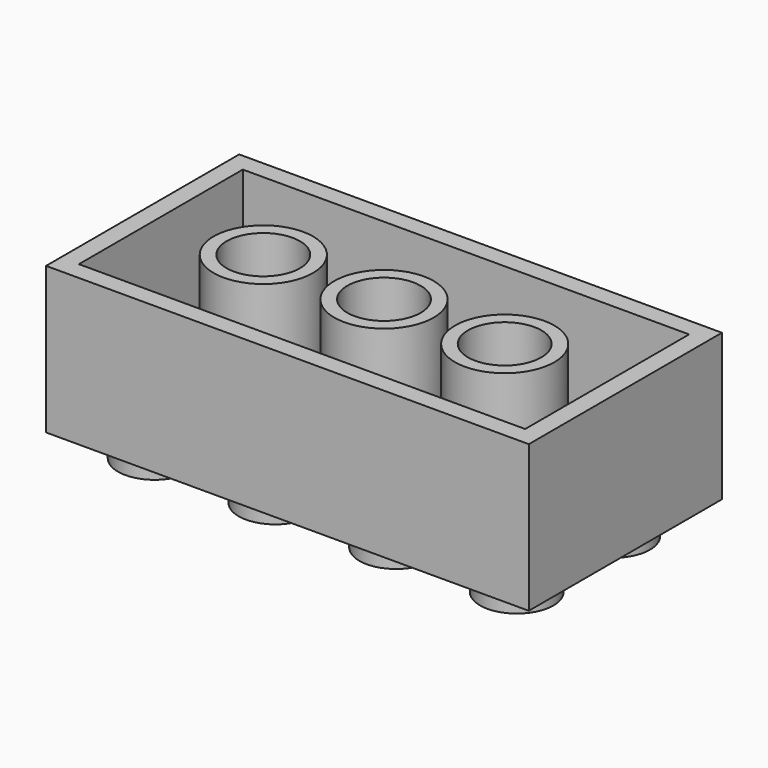
from build123d import *

# Parameters (mm, degrees)
F0_R     = 2.4003
F1_DEPTH = 9.6012
F2_DEPTH = 1.8034
F3_T     = -1.1938
F4_R     = 3.2512
F4_R_2   = 2.4003
F5_DEPTH = 9.6012


# Not quite as in the source:
# - a feature names something its author has since deleted; it is built from what else it names


with BuildPart() as f1:
    # F0 (on Top) → F1 (new body)
    with BuildSketch(Plane.XY):
        Polygon((-11.8491, 16.497923825), (-11.8491, 8.598523825), (-11.8491, 0.699123825), (-3.9497, 0.699123825), (3.9497, 0.699123825), (11.8491, 0.699123825), (19.7485, 0.699123825), (19.7485, 8.598523825), (19.7485, 16.497923825), (11.8491, 16.497923825), (3.9497, 16.497923825), (-3.9497, 16.497923825), align=None)
        with Locations((-7.8994, 4.648823825)):
            Circle(F0_R, mode=Mode.SUBTRACT)
        with Locations((0, 4.648823825)):
            Circle(F0_R, mode=Mode.SUBTRACT)
        with Locations((7.8994, 4.648823825)):
            Circle(F0_R, mode=Mode.SUBTRACT)
        with Locations((15.7988, 4.648823825)):
            Circle(F0_R, mode=Mode.SUBTRACT)
        with Locations((-7.8994, 12.548223825)):
            Circle(F0_R, mode=Mode.SUBTRACT)
        with Locations((0, 12.548223825)):
            Circle(F0_R, mode=Mode.SUBTRACT)
        with Locations((7.8994, 12.548223825)):
            Circle(F0_R, mode=Mode.SUBTRACT)
        with Locations((15.7988, 12.548223825)):
            Circle(F0_R, mode=Mode.SUBTRACT)
        with Locations((-7.8994, 4.648823825)):
            Circle(F0_R)
        with Locations((-7.8994, 12.548223825)):
            Circle(F0_R)
        with Locations((0, 4.648823825)):
            Circle(F0_R)
        with Locations((0, 12.548223825)):
            Circle(F0_R)
        with Locations((7.8994, 4.648823825)):
            Circle(F0_R)
        with Locations((15.7988, 4.648823825)):
            Circle(F0_R)
        with Locations((15.7988, 12.548223825)):
            Circle(F0_R)
        with Locations((7.8994, 12.548223825)):
            Circle(F0_R)
    extrude(amount=F1_DEPTH)

    # F3
    f3_openings = [f1.faces().sort_by_distance(p)[0] for p in [
        (3.9497, 8.598524, 9.6012),
    ]]
    offset(amount=F3_T, openings=f3_openings)

    # F4 (on face) → F5 (join)
    with BuildSketch(Plane.XY.offset(9.6012)):
        with Locations((-3.9497, 8.598523825)):
            Circle(F4_R)
        with Locations((-3.9497, 8.598523825)):
            Circle(F4_R_2, mode=Mode.SUBTRACT)
        with Locations((3.9497, 8.598523825)):
            Circle(F4_R)
        with Locations((3.9497, 8.598523825)):
            Circle(F4_R_2, mode=Mode.SUBTRACT)
        with Locations((11.8491, 8.598523825)):
            Circle(F4_R)
        with Locations((11.8491, 8.598523825)):
            Circle(F4_R_2, mode=Mode.SUBTRACT)
    extrude(amount=-F5_DEPTH)


with BuildPart() as f2:
    # F0 (on Top) → F2 (new body)
    with BuildSketch(Plane.XY):
        with Locations((-7.8994, 4.648823825)):
            Circle(F0_R)
    extrude(amount=-F2_DEPTH)


with BuildPart() as f2b:
    # F0 (on Top) → F2, piece 2 (new body)
    with BuildSketch(Plane.XY):
        with Locations((0, 4.648823825)):
            Circle(F0_R)
    extrude(amount=-F2_DEPTH)


with BuildPart() as f2c:
    # F0 (on Top) → F2, piece 3 (new body)
    with BuildSketch(Plane.XY):
        with Locations((0, 12.548223825)):
            Circle(F0_R)
    extrude(amount=-F2_DEPTH)


with BuildPart() as f2d:
    # F0 (on Top) → F2, piece 4 (new body)
    with BuildSketch(Plane.XY):
        with Locations((-7.8994, 12.548223825)):
            Circle(F0_R)
    extrude(amount=-F2_DEPTH)


with BuildPart() as f2e:
    # F0 (on Top) → F2, piece 5 (new body)
    with BuildSketch(Plane.XY):
        with Locations((7.8994, 4.648823825)):
            Circle(F0_R)
    extrude(amount=-F2_DEPTH)


with BuildPart() as f2f:
    # F0 (on Top) → F2, piece 6 (new body)
    with BuildSketch(Plane.XY):
        with Locations((7.8994, 12.548223825)):
            Circle(F0_R)
    extrude(amount=-F2_DEPTH)


with BuildPart() as f2g:
    # F0 (on Top) → F2, piece 7 (new body)
    with BuildSketch(Plane.XY):
        with Locations((15.7988, 4.648823825)):
            Circle(F0_R)
    extrude(amount=-F2_DEPTH)


with BuildPart() as f2h:
    # F0 (on Top) → F2, piece 8 (new body)
    with BuildSketch(Plane.XY):
        with Locations((15.7988, 12.548223825)):
            Circle(F0_R)
    extrude(amount=-F2_DEPTH)


solid = Compound([f1.part, f2.part, f2b.part, f2c.part, f2d.part, f2e.part, f2f.part, f2g.part, f2h.part])
